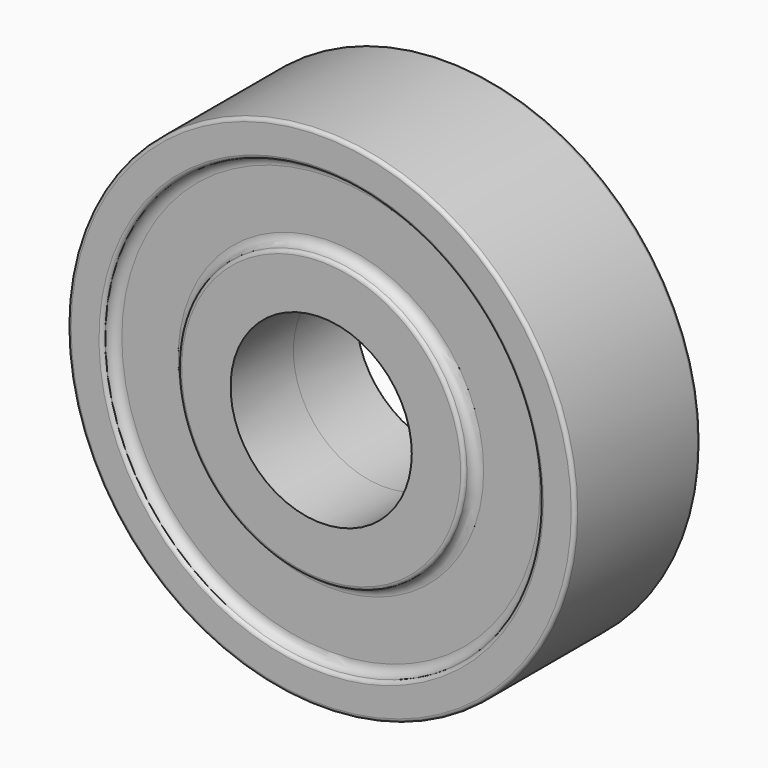
from build123d import *

# Parameters (mm, degrees)
F0_R          = 21
F0_R_2        = 7.5
F1_DEPTH      = 6.5
F1_DEPTH_BACK = 6.5
F2_R          = 18.1
F2_R_2        = 11.85
F3_DEPTH      = 1
F4_R          = 0.8
F5_R          = 0.3


# Not quite as in the source:
# - a pattern or mirror of a feature is missing from the dataset's text; its kind, count and spacing are read off the source's solid


with BuildPart() as f1:
    # F0 (on Front) → F1 (new body, two sides)
    with BuildSketch(Plane.XZ) as f1_sk:
        Circle(F0_R)
        Circle(F0_R_2, mode=Mode.SUBTRACT)
    extrude(amount=F1_DEPTH)
    extrude(f1_sk.sketch, amount=-F1_DEPTH_BACK)

    # F2 (on face) → F3 (cut)
    with BuildSketch(Plane.XZ.offset(6.5)):
        Circle(F2_R)
        Circle(F2_R_2, mode=Mode.SUBTRACT)
    f3 = extrude(amount=-F3_DEPTH, mode=Mode.SUBTRACT)

    # F3_copies: F3 across plane
    add(f3.mirror(Plane.ZX), mode=Mode.SUBTRACT)

    # F4
    f4_edges = [f1.edges().sort_by_distance(p)[0] for p in [
        (-11.85, -5.5, 0),
        (-18.1, -5.5, 0),
        (-18.1, 5.5, 0),
        (-11.85, 5.5, 0),
    ]]
    fillet(f4_edges, radius=F4_R)

    # F5
    f5_edges = [f1.edges().sort_by_distance(p)[0] for p in [
        (-18.1, -6.5, 0),
        (-21, -6.5, 0),
        (-11.85, -6.5, 0),
        (-21, 6.5, 0),
        (-18.1, 6.5, 0),
        (-11.85, 6.5, 0),
    ]]
    fillet(f5_edges, radius=F5_R)


solid = f1.part
